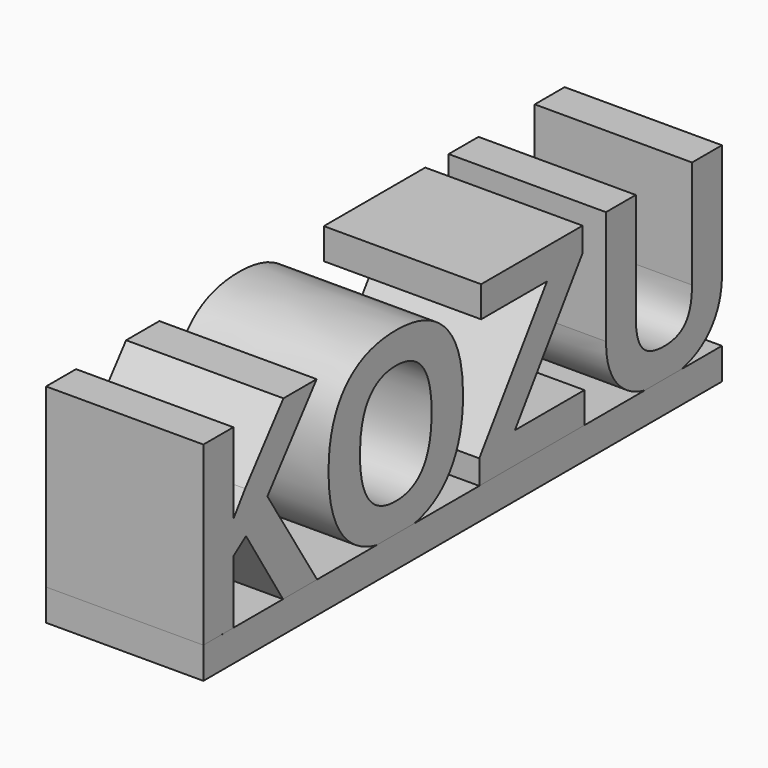
from build123d import *

# Parameters (mm, degrees)
F0_TEXT_SIZE = 39.9435482298
F1_DEPTH     = 25.4
F2_W         = 25.4001040012
F2_H         = 104.6583337387
F3_DEPTH     = 5.08


# Not quite as in the source:
# - Text() gives the source's letters only with a copy of the font that has no kerning and outlines rounded to 1/6400 em; it was checked with that copy


with BuildPart() as f1:
    # F0 (on Right) → F1 (new body)
    with BuildSketch(Plane.YZ):
        with Locations((-41.2033051252, -12.0752416551)):
            Text('KOZU', F0_TEXT_SIZE, font='Open Sans', font_style=FontStyle.BOLD, text_align=(TextAlign.LEFT, TextAlign.BOTTOM))
    extrude(amount=F1_DEPTH)


with BuildPart() as f3:
    # F2 (on face) → F3 (new body)
    with BuildSketch(Plane(origin=(0, 0, -12.0752416551), x_dir=(1, 0, 0), z_dir=(0, 0, -1))):
        with Locations((12.7000520006, -14.7145399054)):
            Rectangle(F2_W, F2_H)
    extrude(amount=F3_DEPTH)


solid = Compound([f1.part, f3.part])
